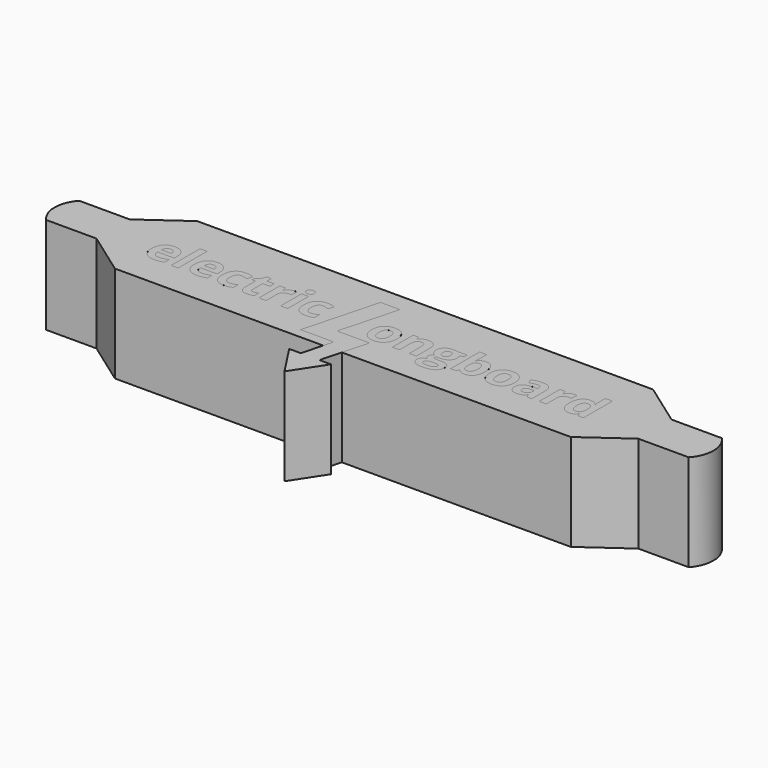
from build123d import *

# Parameters (mm, degrees)
F0_W         = 1.8341714676
F0_H         = 9.3594709833
F0_H_2       = 6.7246538383
F1_DEPTH     = 25
F2_DEPTH     = 25
F3_DEPTH     = 25
F4_DEPTH     = 25
F0_TEXT_SIZE = 12.3176258057
F5_DEPTH     = 25


# Not quite as in the source:
# - Text() gives the source's letters only with a copy of the font that has no kerning and outlines rounded to 1/6400 em; it was checked with that copy


with BuildPart() as f1:
    # F0 (on Top) → F1 (new body)
    with BuildSketch(Plane.XY):
        with BuildLine():
            Line((-5.1384238204, -5.5999981016), (0.0308822297, 13.7858465301))
            Line((0.0308822297, 13.7858465301), (5.042217245, 13.7858465301))
            Line((5.042217245, 13.7858465301), (0.9836744241, -1.434432516))
            Line((0.9836744241, -1.434432516), (9.3703576215, -1.434432516))
            Line((9.3703576215, -1.434432516), (7.5798184046, -8.1492825808))
            Line((7.5798184046, -8.1492825808), (66.7315653023, -8.1492825808))
            Line((66.7315653023, -8.1492825808), (77.8353717101, -0.2207219492))
            Line((77.8353717101, -0.2207219492), (90.8519435273, -0.2207219492))
            ThreePointArc((90.8519435273, -0.2207219492), (92.9463269801, 5.1369656589), (90.8519435273, 10.494653267))
            Line((90.8519435273, 10.494653267), (77.8353717101, 10.494653267))
            Line((77.8353717101, 10.494653267), (66.7315653023, 18.4232138986))
            Line((66.7315653023, 18.4232138986), (-51.0450346977, 18.4232138986))
            Line((-51.0450346977, 18.4232138986), (-62.1488411056, 10.494653267))
            Line((-62.1488411056, 10.494653267), (-75.1654129228, 10.494653267))
            ThreePointArc((-75.1654129228, 10.494653267), (-77.2597963755, 5.1369656589), (-75.1654129228, -0.2207219492))
            Line((-75.1654129228, -0.2207219492), (-62.1488411056, -0.2207219492))
            Line((-62.1488411056, -0.2207219492), (-51.0450346977, -8.1492825808))
            Line((-51.0450346977, -8.1492825808), (2.7661361966, -8.1492825808))
            Line((2.7661361966, -8.1492825808), (3.4459121843, -5.5999981016))
            Line((3.4459121843, -5.5999981016), (-5.1384238204, -5.5999981016))
        make_face()
        with BuildLine():
            add(Edge.make_bspline(
                [(-45.9638463726, -0.0038492581), (-46.5104410177, -0.121251629), (-47.2995389209, -0.121251629)],
                knots=[0, 0, 0, 1, 1, 1], degree=2))
            add(Edge.make_bspline(
                [(-47.2995389209, -0.121251629), (-48.922001195, -0.121251629), (-49.8361999853, 0.7756255)],
                knots=[0, 0, 0, 1, 1, 1], degree=2))
            add(Edge.make_bspline(
                [(-49.8361999853, 0.7756255), (-50.7503987756, 1.6725026289), (-50.7503987756, 3.3142111934)],
                knots=[0, 0, 0, 1, 1, 1], degree=2))
            add(Edge.make_bspline(
                [(-50.7503987756, 3.3142111934), (-50.7503987756, 5.0040354836), (-49.9054866305, 5.9268951045)],
                knots=[0, 0, 0, 1, 1, 1], degree=2))
            add(Edge.make_bspline(
                [(-49.9054866305, 5.9268951045), (-49.0605744853, 6.8497547254), (-47.5689869854, 6.8497547254)],
                knots=[0, 0, 0, 1, 1, 1], degree=2))
            add(Edge.make_bspline(
                [(-47.5689869854, 6.8497547254), (-46.1447615016, 6.8497547254), (-45.3508520259, 6.0385235884)],
                knots=[0, 0, 0, 1, 1, 1], degree=2))
            add(Edge.make_bspline(
                [(-45.3508520259, 6.0385235884), (-44.5569425501, 5.2272924513), (-44.5569425501, 3.7953684514)],
                knots=[0, 0, 0, 1, 1, 1], degree=2))
            Line((-44.5569425501, 3.7953684514), (-44.5569425501, 2.9042652095))
            Line((-44.5569425501, 2.9042652095), (-48.8931317595, 2.9042652095))
            add(Edge.make_bspline(
                [(-48.8931317595, 2.9042652095), (-48.862337695, 2.1228658225), (-48.4292961628, 1.6840504031)],
                knots=[0, 0, 0, 1, 1, 1], degree=2))
            add(Edge.make_bspline(
                [(-48.4292961628, 1.6840504031), (-47.9962546306, 1.2452349838), (-47.2148552435, 1.2452349838)],
                knots=[0, 0, 0, 1, 1, 1], degree=2))
            add(Edge.make_bspline(
                [(-47.2148552435, 1.2452349838), (-46.6066724694, 1.2452349838), (-46.0658517113, 1.3712981854)],
                knots=[0, 0, 0, 1, 1, 1], degree=2))
            add(Edge.make_bspline(
                [(-46.0658517113, 1.3712981854), (-45.5250309533, 1.497361387), (-44.9360944694, 1.7745079676)],
                knots=[0, 0, 0, 1, 1, 1], degree=2))
            Line((-44.9360944694, 1.7745079676), (-44.9360944694, 0.3541317419))
            add(Edge.make_bspline(
                [(-44.9360944694, 0.3541317419), (-45.4172517275, 0.1135531129), (-45.9638463726, -0.0038492581)],
                knots=[0, 0, 0, 1, 1, 1], degree=2))
        make_face(mode=Mode.SUBTRACT)
        with BuildLine():
            add(Edge.make_bspline(
                [(-34.9280235023, -0.0038492581), (-35.4746181474, -0.121251629), (-36.2637160506, -0.121251629)],
                knots=[0, 0, 0, 1, 1, 1], degree=2))
            add(Edge.make_bspline(
                [(-36.2637160506, -0.121251629), (-37.8861783247, -0.121251629), (-38.800377115, 0.7756255)],
                knots=[0, 0, 0, 1, 1, 1], degree=2))
            add(Edge.make_bspline(
                [(-38.800377115, 0.7756255), (-39.7145759052, 1.6725026289), (-39.7145759052, 3.3142111934)],
                knots=[0, 0, 0, 1, 1, 1], degree=2))
            add(Edge.make_bspline(
                [(-39.7145759052, 3.3142111934), (-39.7145759052, 5.0040354836), (-38.8696637601, 5.9268951045)],
                knots=[0, 0, 0, 1, 1, 1], degree=2))
            add(Edge.make_bspline(
                [(-38.8696637601, 5.9268951045), (-38.024751615, 6.8497547254), (-36.5331641151, 6.8497547254)],
                knots=[0, 0, 0, 1, 1, 1], degree=2))
            add(Edge.make_bspline(
                [(-36.5331641151, 6.8497547254), (-35.1089386313, 6.8497547254), (-34.3150291556, 6.0385235884)],
                knots=[0, 0, 0, 1, 1, 1], degree=2))
            add(Edge.make_bspline(
                [(-34.3150291556, 6.0385235884), (-33.5211196798, 5.2272924513), (-33.5211196798, 3.7953684514)],
                knots=[0, 0, 0, 1, 1, 1], degree=2))
            Line((-33.5211196798, 3.7953684514), (-33.5211196798, 2.9042652095))
            Line((-33.5211196798, 2.9042652095), (-37.8573088892, 2.9042652095))
            add(Edge.make_bspline(
                [(-37.8573088892, 2.9042652095), (-37.8265148247, 2.1228658225), (-37.3934732925, 1.6840504031)],
                knots=[0, 0, 0, 1, 1, 1], degree=2))
            add(Edge.make_bspline(
                [(-37.3934732925, 1.6840504031), (-36.9604317602, 1.2452349838), (-36.1790323732, 1.2452349838)],
                knots=[0, 0, 0, 1, 1, 1], degree=2))
            add(Edge.make_bspline(
                [(-36.1790323732, 1.2452349838), (-35.570849599, 1.2452349838), (-35.030028841, 1.3712981854)],
                knots=[0, 0, 0, 1, 1, 1], degree=2))
            add(Edge.make_bspline(
                [(-35.030028841, 1.3712981854), (-34.489208083, 1.497361387), (-33.9002715991, 1.7745079676)],
                knots=[0, 0, 0, 1, 1, 1], degree=2))
            Line((-33.9002715991, 1.7745079676), (-33.9002715991, 0.3541317419))
            add(Edge.make_bspline(
                [(-33.9002715991, 0.3541317419), (-34.3814288572, 0.1135531129), (-34.9280235023, -0.0038492581)],
                knots=[0, 0, 0, 1, 1, 1], degree=2))
        make_face(mode=Mode.SUBTRACT)
        with Locations((-42.1482693164, 4.6797354917)):
            Rectangle(F0_W, F0_H, mode=Mode.SUBTRACT)
        with BuildLine():
            add(Edge.make_bspline(
                [(-28.1533293091, -0.0125100887), (-28.6075417607, -0.121251629), (-29.2984835833, -0.121251629)],
                knots=[0, 0, 0, 1, 1, 1], degree=2))
            add(Edge.make_bspline(
                [(-29.2984835833, -0.121251629), (-32.4375535347, -0.121251629), (-32.4375535347, 3.3257589675)],
                knots=[0, 0, 0, 1, 1, 1], degree=2))
            add(Edge.make_bspline(
                [(-32.4375535347, 3.3257589675), (-32.4375535347, 5.0406034352), (-31.5839805589, 5.9451790803)],
                knots=[0, 0, 0, 1, 1, 1], degree=2))
            add(Edge.make_bspline(
                [(-31.5839805589, 5.9451790803), (-30.7304075832, 6.8497547254), (-29.1368147446, 6.8497547254)],
                knots=[0, 0, 0, 1, 1, 1], degree=2))
            add(Edge.make_bspline(
                [(-29.1368147446, 6.8497547254), (-27.9704895511, 6.8497547254), (-27.0428183576, 6.3936176448)],
                knots=[0, 0, 0, 1, 1, 1], degree=2))
            Line((-27.0428183576, 6.3936176448), (-27.5855637447, 4.9732414191))
            add(Edge.make_bspline(
                [(-27.5855637447, 4.9732414191), (-28.0186052769, 5.148382661), (-28.3910209946, 5.2600111449)],
                knots=[0, 0, 0, 1, 1, 1], degree=2))
            add(Edge.make_bspline(
                [(-28.3910209946, 5.2600111449), (-28.7634367123, 5.3716396287), (-29.1368147446, 5.3716396287)],
                knots=[0, 0, 0, 1, 1, 1], degree=2))
            add(Edge.make_bspline(
                [(-29.1368147446, 5.3716396287), (-30.5687387445, 5.3716396287), (-30.5687387445, 3.3373067417)],
                knots=[0, 0, 0, 1, 1, 1], degree=2))
            add(Edge.make_bspline(
                [(-30.5687387445, 3.3373067417), (-30.5687387445, 1.3645619838), (-29.1368147446, 1.3645619838)],
                knots=[0, 0, 0, 1, 1, 1], degree=2))
            add(Edge.make_bspline(
                [(-29.1368147446, 1.3645619838), (-28.6075417607, 1.3645619838), (-28.1562162527, 1.5060222177)],
                knots=[0, 0, 0, 1, 1, 1], degree=2))
            add(Edge.make_bspline(
                [(-28.1562162527, 1.5060222177), (-27.7048907446, 1.6474824515), (-27.2545275511, 1.9496492096)],
                knots=[0, 0, 0, 1, 1, 1], degree=2))
            Line((-27.2545275511, 1.9496492096), (-27.2545275511, 0.3791519193))
            add(Edge.make_bspline(
                [(-27.2545275511, 0.3791519193), (-27.6991168575, 0.0962314516), (-28.1533293091, -0.0125100887)],
                knots=[0, 0, 0, 1, 1, 1], degree=2))
        make_face(mode=Mode.SUBTRACT)
        with BuildLine():
            add(Edge.make_bspline(
                [(-23.4437620675, 1.5281554515), (-23.2243543578, 1.3414664354), (-22.8625240998, 1.3414664354)],
                knots=[0, 0, 0, 1, 1, 1], degree=2))
            add(Edge.make_bspline(
                [(-22.8625240998, 1.3414664354), (-22.3813668417, 1.3414664354), (-21.7077466805, 1.5512509999)],
                knots=[0, 0, 0, 1, 1, 1], degree=2))
            Line((-21.7077466805, 1.5512509999), (-21.7077466805, 0.1866890161))
            add(Edge.make_bspline(
                [(-21.7077466805, 0.1866890161), (-22.3929146159, -0.121251629), (-23.3917970836, -0.121251629)],
                knots=[0, 0, 0, 1, 1, 1], degree=2))
            add(Edge.make_bspline(
                [(-23.3917970836, -0.121251629), (-24.49268489, -0.121251629), (-24.9950130674, 0.4359284758)],
                knots=[0, 0, 0, 1, 1, 1], degree=2))
            add(Edge.make_bspline(
                [(-24.9950130674, 0.4359284758), (-25.4973412448, 0.9931085806), (-25.4973412448, 2.1055441612)],
                knots=[0, 0, 0, 1, 1, 1], degree=2))
            Line((-25.4973412448, 2.1055441612), (-25.4973412448, 5.3466194513))
            Line((-25.4973412448, 5.3466194513), (-26.3749720834, 5.3466194513))
            Line((-26.3749720834, 5.3466194513), (-26.3749720834, 6.1222449513))
            Line((-26.3749720834, 6.1222449513), (-25.3645418416, 6.7362016125))
            Line((-25.3645418416, 6.7362016125), (-24.8352688577, 8.1565778382))
            Line((-24.8352688577, 8.1565778382), (-23.6631697771, 8.1565778382))
            Line((-23.6631697771, 8.1565778382), (-23.6631697771, 6.7246538383))
            Line((-23.6631697771, 6.7246538383), (-21.7808825837, 6.7246538383))
            Line((-21.7808825837, 6.7246538383), (-21.7808825837, 5.3466194513))
            Line((-21.7808825837, 5.3466194513), (-23.6631697771, 5.3466194513))
            Line((-23.6631697771, 5.3466194513), (-23.6631697771, 2.1055441612))
            add(Edge.make_bspline(
                [(-23.6631697771, 2.1055441612), (-23.6631697771, 1.7148444676), (-23.4437620675, 1.5281554515)],
                knots=[0, 0, 0, 1, 1, 1], degree=2))
        make_face(mode=Mode.SUBTRACT)
        with BuildLine():
            add(Edge.make_bspline(
                [(-17.7535963339, 6.5042838141), (-17.2214364065, 6.8497547254), (-16.5959319711, 6.8497547254)],
                knots=[0, 0, 0, 1, 1, 1], degree=2))
            add(Edge.make_bspline(
                [(-16.5959319711, 6.8497547254), (-16.2225539389, 6.8497547254), (-15.9762014227, 6.7958651125)],
                knots=[0, 0, 0, 1, 1, 1], degree=2))
            Line((-15.9762014227, 6.7958651125), (-16.1147747131, 5.0771713868))
            add(Edge.make_bspline(
                [(-16.1147747131, 5.0771713868), (-16.3380316808, 5.1368348868), (-16.6555954711, 5.1368348868)],
                knots=[0, 0, 0, 1, 1, 1], degree=2))
            add(Edge.make_bspline(
                [(-16.6555954711, 5.1368348868), (-17.5332263098, 5.1368348868), (-18.0240067129, 4.6855093788)],
                knots=[0, 0, 0, 1, 1, 1], degree=2))
            add(Edge.make_bspline(
                [(-18.0240067129, 4.6855093788), (-18.5147871161, 4.2341838707), (-18.5147871161, 3.4219904192)],
                knots=[0, 0, 0, 1, 1, 1], degree=2))
            Line((-18.5147871161, 3.4219904192), (-18.5147871161, 0))
            Line((-18.5147871161, 0), (-20.3489585838, 0))
            Line((-20.3489585838, 0), (-20.3489585838, 6.7246538383))
            Line((-20.3489585838, 6.7246538383), (-18.9593764226, 6.7246538383))
            Line((-18.9593764226, 6.7246538383), (-18.688003729, 5.5929719674))
            Line((-18.688003729, 5.5929719674), (-18.5994707936, 5.5929719674))
            add(Edge.make_bspline(
                [(-18.5994707936, 5.5929719674), (-18.2857562613, 6.1588129029), (-17.7535963339, 6.5042838141)],
                knots=[0, 0, 0, 1, 1, 1], degree=2))
        make_face(mode=Mode.SUBTRACT)
        with Locations((-13.8389008825, 3.3623269192)):
            Rectangle(F0_W, F0_H_2, mode=Mode.SUBTRACT)
        with BuildLine():
            add(Edge.make_bspline(
                [(-7.1209832458, -0.0125100887), (-7.5751956974, -0.121251629), (-8.26613752, -0.121251629)],
                knots=[0, 0, 0, 1, 1, 1], degree=2))
            add(Edge.make_bspline(
                [(-8.26613752, -0.121251629), (-11.4052074714, -0.121251629), (-11.4052074714, 3.3257589675)],
                knots=[0, 0, 0, 1, 1, 1], degree=2))
            add(Edge.make_bspline(
                [(-11.4052074714, 3.3257589675), (-11.4052074714, 5.0406034352), (-10.5516344956, 5.9451790803)],
                knots=[0, 0, 0, 1, 1, 1], degree=2))
            add(Edge.make_bspline(
                [(-10.5516344956, 5.9451790803), (-9.6980615199, 6.8497547254), (-8.1044686813, 6.8497547254)],
                knots=[0, 0, 0, 1, 1, 1], degree=2))
            add(Edge.make_bspline(
                [(-8.1044686813, 6.8497547254), (-6.9381434878, 6.8497547254), (-6.0104722943, 6.3936176448)],
                knots=[0, 0, 0, 1, 1, 1], degree=2))
            Line((-6.0104722943, 6.3936176448), (-6.5532176814, 4.9732414191))
            add(Edge.make_bspline(
                [(-6.5532176814, 4.9732414191), (-6.9862592136, 5.148382661), (-7.3586749313, 5.2600111449)],
                knots=[0, 0, 0, 1, 1, 1], degree=2))
            add(Edge.make_bspline(
                [(-7.3586749313, 5.2600111449), (-7.731090649, 5.3716396287), (-8.1044686813, 5.3716396287)],
                knots=[0, 0, 0, 1, 1, 1], degree=2))
            add(Edge.make_bspline(
                [(-8.1044686813, 5.3716396287), (-9.5363926812, 5.3716396287), (-9.5363926812, 3.3373067417)],
                knots=[0, 0, 0, 1, 1, 1], degree=2))
            add(Edge.make_bspline(
                [(-9.5363926812, 3.3373067417), (-9.5363926812, 1.3645619838), (-8.1044686813, 1.3645619838)],
                knots=[0, 0, 0, 1, 1, 1], degree=2))
            add(Edge.make_bspline(
                [(-8.1044686813, 1.3645619838), (-7.5751956974, 1.3645619838), (-7.1238701894, 1.5060222177)],
                knots=[0, 0, 0, 1, 1, 1], degree=2))
            add(Edge.make_bspline(
                [(-7.1238701894, 1.5060222177), (-6.6725446814, 1.6474824515), (-6.2221814878, 1.9496492096)],
                knots=[0, 0, 0, 1, 1, 1], degree=2))
            Line((-6.2221814878, 1.9496492096), (-6.2221814878, 0.3791519193))
            add(Edge.make_bspline(
                [(-6.2221814878, 0.3791519193), (-6.6667707943, 0.0962314516), (-7.1209832458, -0.0125100887)],
                knots=[0, 0, 0, 1, 1, 1], degree=2))
        make_face(mode=Mode.SUBTRACT)
        with BuildLine():
            add(Edge.make_bspline(
                [(-13.836013939, 7.5599428383), (-14.8348964067, 7.5599428383), (-14.8348964067, 8.4625938543)],
                knots=[0, 0, 0, 1, 1, 1], degree=2))
            add(Edge.make_bspline(
                [(-14.8348964067, 8.4625938543), (-14.8348964067, 9.3594709833), (-13.836013939, 9.3594709833)],
                knots=[0, 0, 0, 1, 1, 1], degree=2))
            add(Edge.make_bspline(
                [(-13.836013939, 9.3594709833), (-12.8371314713, 9.3594709833), (-12.8371314713, 8.4625938543)],
                knots=[0, 0, 0, 1, 1, 1], degree=2))
            add(Edge.make_bspline(
                [(-12.8371314713, 8.4625938543), (-12.8371314713, 8.0353262092), (-13.086370931, 7.7976345237)],
                knots=[0, 0, 0, 1, 1, 1], degree=2))
            add(Edge.make_bspline(
                [(-13.086370931, 7.7976345237), (-13.3356103906, 7.5599428383), (-13.836013939, 7.5599428383)],
                knots=[0, 0, 0, 1, 1, 1], degree=2))
        make_face(mode=Mode.SUBTRACT)
        with BuildLine():
            Line((25.7141219699, 6.7246538383), (28.0602447601, 6.7246538383))
            Line((28.0602447601, 6.7246538383), (28.0602447601, 5.7912087577))
            Line((28.0602447601, 5.7912087577), (27.0074726795, 5.5217606932))
            add(Edge.make_bspline(
                [(27.0074726795, 5.5217606932), (27.2961670344, 5.0694728707), (27.2961670344, 4.5113304514)],
                knots=[0, 0, 0, 1, 1, 1], degree=2))
            add(Edge.make_bspline(
                [(27.2961670344, 4.5113304514), (27.2961670344, 3.4277643063), (26.5407501392, 2.8234307902)],
                knots=[0, 0, 0, 1, 1, 1], degree=2))
            add(Edge.make_bspline(
                [(26.5407501392, 2.8234307902), (25.7853332441, 2.2190972741), (24.4457914378, 2.2190972741)],
                knots=[0, 0, 0, 1, 1, 1], degree=2))
            Line((24.4457914378, 2.2190972741), (24.1147552442, 2.2383435644))
            Line((24.1147552442, 2.2383435644), (23.8433825507, 2.2672129999))
            add(Edge.make_bspline(
                [(23.8433825507, 2.2672129999), (23.560462083, 2.0516545483), (23.560462083, 1.7860557418)],
                knots=[0, 0, 0, 1, 1, 1], degree=2))
            add(Edge.make_bspline(
                [(23.560462083, 1.7860557418), (23.560462083, 1.3895821612), (24.5708923248, 1.3895821612)],
                knots=[0, 0, 0, 1, 1, 1], degree=2))
            Line((24.5708923248, 1.3895821612), (25.7141219699, 1.3895821612))
            add(Edge.make_bspline(
                [(25.7141219699, 1.3895821612), (26.8207836634, 1.3895821612), (27.4010593166, 0.9141987903)],
                knots=[0, 0, 0, 1, 1, 1], degree=2))
            add(Edge.make_bspline(
                [(27.4010593166, 0.9141987903), (27.9813349698, 0.4388154193), (27.9813349698, -0.481157258)],
                knots=[0, 0, 0, 1, 1, 1], degree=2))
            add(Edge.make_bspline(
                [(27.9813349698, -0.481157258), (27.9813349698, -1.6609548547), (26.9978495344, -2.3105171531)],
                knots=[0, 0, 0, 1, 1, 1], degree=2))
            add(Edge.make_bspline(
                [(26.9978495344, -2.3105171531), (26.014364099, -2.9600794514), (24.1744187442, -2.9600794514)],
                knots=[0, 0, 0, 1, 1, 1], degree=2))
            add(Edge.make_bspline(
                [(24.1744187442, -2.9600794514), (22.7675149217, -2.9600794514), (22.0246081153, -2.4692990482)],
                knots=[0, 0, 0, 1, 1, 1], degree=2))
            add(Edge.make_bspline(
                [(22.0246081153, -2.4692990482), (21.2817013089, -1.978518645), (21.2817013089, -1.0951139193)],
                knots=[0, 0, 0, 1, 1, 1], degree=2))
            add(Edge.make_bspline(
                [(21.2817013089, -1.0951139193), (21.2817013089, -0.4869311451), (21.6608532282, -0.0779474758)],
                knots=[0, 0, 0, 1, 1, 1], degree=2))
            add(Edge.make_bspline(
                [(21.6608532282, -0.0779474758), (22.0400051476, 0.3310361935), (22.7732888088, 0.5061774355)],
                knots=[0, 0, 0, 1, 1, 1], degree=2))
            add(Edge.make_bspline(
                [(22.7732888088, 0.5061774355), (22.4903683411, 0.6255044354), (22.2796214621, 0.898801758)],
                knots=[0, 0, 0, 1, 1, 1], degree=2))
            add(Edge.make_bspline(
                [(22.2796214621, 0.898801758), (22.0688745831, 1.1720990806), (22.0688745831, 1.4800397257)],
                knots=[0, 0, 0, 1, 1, 1], degree=2))
            add(Edge.make_bspline(
                [(22.0688745831, 1.4800397257), (22.0688745831, 1.8649655321), (22.2911692363, 2.1199788789)],
                knots=[0, 0, 0, 1, 1, 1], degree=2))
            add(Edge.make_bspline(
                [(22.2911692363, 2.1199788789), (22.5134638895, 2.3749922257), (22.9349576475, 2.6232693708)],
                knots=[0, 0, 0, 1, 1, 1], degree=2))
            add(Edge.make_bspline(
                [(22.9349576475, 2.6232693708), (22.4056846637, 2.8503755966), (22.0958193895, 3.3555907175)],
                knots=[0, 0, 0, 1, 1, 1], degree=2))
            add(Edge.make_bspline(
                [(22.0958193895, 3.3555907175), (21.7859541153, 3.8608058385), (21.7859541153, 4.547898403)],
                knots=[0, 0, 0, 1, 1, 1], degree=2))
            add(Edge.make_bspline(
                [(21.7859541153, 4.547898403), (21.7859541153, 5.6468615803), (22.5019161153, 6.2483081529)],
                knots=[0, 0, 0, 1, 1, 1], degree=2))
            add(Edge.make_bspline(
                [(22.5019161153, 6.2483081529), (23.2178781152, 6.8497547254), (24.5477967765, 6.8497547254)],
                knots=[0, 0, 0, 1, 1, 1], degree=2))
            add(Edge.make_bspline(
                [(24.5477967765, 6.8497547254), (24.8307172442, 6.8497547254), (25.2185299942, 6.7987520561)],
                knots=[0, 0, 0, 1, 1, 1], degree=2))
            add(Edge.make_bspline(
                [(25.2185299942, 6.7987520561), (25.6063427441, 6.7477493867), (25.7141219699, 6.7246538383)],
                knots=[0, 0, 0, 1, 1, 1], degree=2))
        make_face(mode=Mode.SUBTRACT)
        with BuildLine():
            add(Edge.make_bspline(
                [(12.1993769062, 5.2205562497), (12.5958504868, 4.432420661), (12.5958504868, 3.3738746934)],
                knots=[0, 0, 0, 1, 1, 1], degree=2))
            add(Edge.make_bspline(
                [(12.5958504868, 3.3738746934), (12.5958504868, 1.7321661289), (11.7297674224, 0.80545725)],
                knots=[0, 0, 0, 1, 1, 1], degree=2))
            add(Edge.make_bspline(
                [(11.7297674224, 0.80545725), (10.8636843579, -0.121251629), (9.3182072451, -0.121251629)],
                knots=[0, 0, 0, 1, 1, 1], degree=2))
            add(Edge.make_bspline(
                [(9.3182072451, -0.121251629), (8.3501188419, -0.121251629), (7.6100989791, 0.3031290726)],
                knots=[0, 0, 0, 1, 1, 1], degree=2))
            add(Edge.make_bspline(
                [(7.6100989791, 0.3031290726), (6.8700791162, 0.7275097742), (6.4736055356, 1.5214192499)],
                knots=[0, 0, 0, 1, 1, 1], degree=2))
            add(Edge.make_bspline(
                [(6.4736055356, 1.5214192499), (6.077131955, 2.3153287257), (6.077131955, 3.3738746934)],
                knots=[0, 0, 0, 1, 1, 1], degree=2))
            add(Edge.make_bspline(
                [(6.077131955, 3.3738746934), (6.077131955, 5.0213571449), (6.9364788178, 5.9355559351)],
                knots=[0, 0, 0, 1, 1, 1], degree=2))
            add(Edge.make_bspline(
                [(6.9364788178, 5.9355559351), (7.7958256807, 6.8497547254), (9.3547751967, 6.8497547254)],
                knots=[0, 0, 0, 1, 1, 1], degree=2))
            add(Edge.make_bspline(
                [(9.3547751967, 6.8497547254), (10.3228635999, 6.8497547254), (11.0628834627, 6.4292232819)],
                knots=[0, 0, 0, 1, 1, 1], degree=2))
            add(Edge.make_bspline(
                [(11.0628834627, 6.4292232819), (11.8029033256, 6.0086918384), (12.1993769062, 5.2205562497)],
                knots=[0, 0, 0, 1, 1, 1], degree=2))
        make_face(mode=Mode.SUBTRACT)
        with BuildLine():
            Line((20.3193867928, 4.3843049352), (20.3193867928, 0))
            Line((20.3193867928, 0), (18.4852153252, 0))
            Line((18.4852153252, 0), (18.4852153252, 3.9281678546))
            add(Edge.make_bspline(
                [(18.4852153252, 3.9281678546), (18.4852153252, 4.6556776288), (18.2263527204, 5.0194325158)],
                knots=[0, 0, 0, 1, 1, 1], degree=2))
            add(Edge.make_bspline(
                [(18.2263527204, 5.0194325158), (17.9674901156, 5.3831874029), (17.4016491801, 5.3831874029)],
                knots=[0, 0, 0, 1, 1, 1], degree=2))
            add(Edge.make_bspline(
                [(17.4016491801, 5.3831874029), (16.6317975672, 5.3831874029), (16.2892135995, 4.8693114513)],
                knots=[0, 0, 0, 1, 1, 1], degree=2))
            add(Edge.make_bspline(
                [(16.2892135995, 4.8693114513), (15.9466296318, 4.3554354997), (15.9466296318, 3.1640901288)],
                knots=[0, 0, 0, 1, 1, 1], degree=2))
            Line((15.9466296318, 3.1640901288), (15.9466296318, 0))
            Line((15.9466296318, 0), (14.1124581642, 0))
            Line((14.1124581642, 0), (14.1124581642, 6.7246538383))
            Line((14.1124581642, 6.7246538383), (15.5135880996, 6.7246538383))
            Line((15.5135880996, 6.7246538383), (15.7599406157, 5.8643446609))
            Line((15.7599406157, 5.8643446609), (15.8619459544, 5.8643446609))
            add(Edge.make_bspline(
                [(15.8619459544, 5.8643446609), (16.1698865995, 6.3512758061), (16.707820414, 6.6005152657)],
                knots=[0, 0, 0, 1, 1, 1], degree=2))
            add(Edge.make_bspline(
                [(16.707820414, 6.6005152657), (17.2457542285, 6.8497547254), (17.9309221639, 6.8497547254)],
                knots=[0, 0, 0, 1, 1, 1], degree=2))
            add(Edge.make_bspline(
                [(17.9309221639, 6.8497547254), (19.1049458736, 6.8497547254), (19.7121663332, 6.2155894593)],
                knots=[0, 0, 0, 1, 1, 1], degree=2))
            add(Edge.make_bspline(
                [(19.7121663332, 6.2155894593), (20.3193867928, 5.5814241932), (20.3193867928, 4.3843049352)],
                knots=[0, 0, 0, 1, 1, 1], degree=2))
        make_face(mode=Mode.SUBTRACT)
        with BuildLine():
            add(Edge.make_bspline(
                [(31.0010779212, 5.8527968868), (31.645828647, 6.8497547254), (32.9083852921, 6.8497547254)],
                knots=[0, 0, 0, 1, 1, 1], degree=2))
            add(Edge.make_bspline(
                [(32.9083852921, 6.8497547254), (34.099730663, 6.8497547254), (34.7733508243, 5.9211212174)],
                knots=[0, 0, 0, 1, 1, 1], degree=2))
            add(Edge.make_bspline(
                [(34.7733508243, 5.9211212174), (35.4469709855, 4.9924877094), (35.4469709855, 3.3738746934)],
                knots=[0, 0, 0, 1, 1, 1], degree=2))
            add(Edge.make_bspline(
                [(35.4469709855, 3.3738746934), (35.4469709855, 1.7090705805), (34.7521799049, 0.7939094758)],
                knots=[0, 0, 0, 1, 1, 1], degree=2))
            add(Edge.make_bspline(
                [(34.7521799049, 0.7939094758), (34.0573888243, -0.121251629), (32.8602695663, -0.121251629)],
                knots=[0, 0, 0, 1, 1, 1], degree=2))
            add(Edge.make_bspline(
                [(32.8602695663, -0.121251629), (31.6746980825, -0.121251629), (31.0010779212, 0.7390575483)],
                knots=[0, 0, 0, 1, 1, 1], degree=2))
            Line((31.0010779212, 0.7390575483), (30.8759770342, 0.7390575483))
            Line((30.8759770342, 0.7390575483), (30.568036389, 0))
            Line((30.568036389, 0), (29.1669064536, 0))
            Line((29.1669064536, 0), (29.1669064536, 9.3594709833))
            Line((29.1669064536, 9.3594709833), (31.0010779212, 9.3594709833))
            Line((31.0010779212, 9.3594709833), (31.0010779212, 7.1807909189))
            add(Edge.make_bspline(
                [(31.0010779212, 7.1807909189), (31.0010779212, 6.766995677), (30.9298666471, 5.8527968868)],
                knots=[0, 0, 0, 1, 1, 1], degree=2))
            Line((30.9298666471, 5.8527968868), (31.0010779212, 5.8527968868))
        make_face(mode=Mode.SUBTRACT)
        with BuildLine():
            add(Edge.make_bspline(
                [(42.6758776302, 5.2205562497), (43.0723512109, 4.432420661), (43.0723512109, 3.3738746934)],
                knots=[0, 0, 0, 1, 1, 1], degree=2))
            add(Edge.make_bspline(
                [(43.0723512109, 3.3738746934), (43.0723512109, 1.7321661289), (42.2062681464, 0.80545725)],
                knots=[0, 0, 0, 1, 1, 1], degree=2))
            add(Edge.make_bspline(
                [(42.2062681464, 0.80545725), (41.3401850819, -0.121251629), (39.7947079691, -0.121251629)],
                knots=[0, 0, 0, 1, 1, 1], degree=2))
            add(Edge.make_bspline(
                [(39.7947079691, -0.121251629), (38.826619566, -0.121251629), (38.0865997031, 0.3031290726)],
                knots=[0, 0, 0, 1, 1, 1], degree=2))
            add(Edge.make_bspline(
                [(38.0865997031, 0.3031290726), (37.3465798402, 0.7275097742), (36.9501062596, 1.5214192499)],
                knots=[0, 0, 0, 1, 1, 1], degree=2))
            add(Edge.make_bspline(
                [(36.9501062596, 1.5214192499), (36.553632679, 2.3153287257), (36.553632679, 3.3738746934)],
                knots=[0, 0, 0, 1, 1, 1], degree=2))
            add(Edge.make_bspline(
                [(36.553632679, 3.3738746934), (36.553632679, 5.0213571449), (37.4129795418, 5.9355559351)],
                knots=[0, 0, 0, 1, 1, 1], degree=2))
            add(Edge.make_bspline(
                [(37.4129795418, 5.9355559351), (38.2723264047, 6.8497547254), (39.8312759207, 6.8497547254)],
                knots=[0, 0, 0, 1, 1, 1], degree=2))
            add(Edge.make_bspline(
                [(39.8312759207, 6.8497547254), (40.7993643239, 6.8497547254), (41.5393841868, 6.4292232819)],
                knots=[0, 0, 0, 1, 1, 1], degree=2))
            add(Edge.make_bspline(
                [(41.5393841868, 6.4292232819), (42.2794040496, 6.0086918384), (42.6758776302, 5.2205562497)],
                knots=[0, 0, 0, 1, 1, 1], degree=2))
        make_face(mode=Mode.SUBTRACT)
        with BuildLine():
            Line((50.1395890169, 0), (48.8597107105, 0))
            Line((48.8597107105, 0), (48.5036543396, 0.9141987903))
            Line((48.5036543396, 0.9141987903), (48.4555386138, 0.9141987903))
            add(Edge.make_bspline(
                [(48.4555386138, 0.9141987903), (47.9936276461, 0.3310361935), (47.5028472429, 0.1048922823)],
                knots=[0, 0, 0, 1, 1, 1], degree=2))
            add(Edge.make_bspline(
                [(47.5028472429, 0.1048922823), (47.0120668397, -0.121251629), (46.2248935655, -0.121251629)],
                knots=[0, 0, 0, 1, 1, 1], degree=2))
            add(Edge.make_bspline(
                [(46.2248935655, -0.121251629), (45.2568051624, -0.121251629), (44.7005873721, 0.4330415322)],
                knots=[0, 0, 0, 1, 1, 1], degree=2))
            add(Edge.make_bspline(
                [(44.7005873721, 0.4330415322), (44.1443695818, 0.9873346935), (44.1443695818, 2.0093127096)],
                knots=[0, 0, 0, 1, 1, 1], degree=2))
            add(Edge.make_bspline(
                [(44.1443695818, 2.0093127096), (44.1443695818, 3.0794064514), (44.8930502753, 3.5875085159)],
                knots=[0, 0, 0, 1, 1, 1], degree=2))
            add(Edge.make_bspline(
                [(44.8930502753, 3.5875085159), (45.6417309688, 4.0956105804), (47.15064013, 4.1495001933)],
                knots=[0, 0, 0, 1, 1, 1], degree=2))
            Line((47.15064013, 4.1495001933), (48.3188899525, 4.1860681449))
            Line((48.3188899525, 4.1860681449), (48.3188899525, 4.4805363868))
            add(Edge.make_bspline(
                [(48.3188899525, 4.4805363868), (48.3188899525, 5.5025144029), (47.271891759, 5.5025144029)],
                knots=[0, 0, 0, 1, 1, 1], degree=2))
            add(Edge.make_bspline(
                [(47.271891759, 5.5025144029), (46.4654721945, 5.5025144029), (45.3761321623, 5.0155832578)],
                knots=[0, 0, 0, 1, 1, 1], degree=2))
            Line((45.3761321623, 5.0155832578), (44.7698740172, 6.2550443545))
            add(Edge.make_bspline(
                [(44.7698740172, 6.2550443545), (45.9304253236, 6.8632271286), (47.3431030332, 6.8632271286)],
                knots=[0, 0, 0, 1, 1, 1], degree=2))
            add(Edge.make_bspline(
                [(47.3431030332, 6.8632271286), (48.6961172428, 6.8632271286), (49.4178531299, 6.2733283303)],
                knots=[0, 0, 0, 1, 1, 1], degree=2))
            add(Edge.make_bspline(
                [(49.4178531299, 6.2733283303), (50.1395890169, 5.6834295319), (50.1395890169, 4.4805363868)],
                knots=[0, 0, 0, 1, 1, 1], degree=2))
            Line((50.1395890169, 4.4805363868), (50.1395890169, 0))
        make_face(mode=Mode.SUBTRACT)
        with BuildLine():
            add(Edge.make_bspline(
                [(54.6249369763, 6.5042838141), (55.1570969037, 6.8497547254), (55.7826013392, 6.8497547254)],
                knots=[0, 0, 0, 1, 1, 1], degree=2))
            add(Edge.make_bspline(
                [(55.7826013392, 6.8497547254), (56.1559793714, 6.8497547254), (56.4023318875, 6.7958651125)],
                knots=[0, 0, 0, 1, 1, 1], degree=2))
            Line((56.4023318875, 6.7958651125), (56.2637585972, 5.0771713868))
            add(Edge.make_bspline(
                [(56.2637585972, 5.0771713868), (56.0405016295, 5.1368348868), (55.7229378392, 5.1368348868)],
                knots=[0, 0, 0, 1, 1, 1], degree=2))
            add(Edge.make_bspline(
                [(55.7229378392, 5.1368348868), (54.8453070005, 5.1368348868), (54.3545265973, 4.6855093788)],
                knots=[0, 0, 0, 1, 1, 1], degree=2))
            add(Edge.make_bspline(
                [(54.3545265973, 4.6855093788), (53.8637461941, 4.2341838707), (53.8637461941, 3.4219904192)],
                knots=[0, 0, 0, 1, 1, 1], degree=2))
            Line((53.8637461941, 3.4219904192), (53.8637461941, 0))
            Line((53.8637461941, 0), (52.0295747265, 0))
            Line((52.0295747265, 0), (52.0295747265, 6.7246538383))
            Line((52.0295747265, 6.7246538383), (53.4191568877, 6.7246538383))
            Line((53.4191568877, 6.7246538383), (53.6905295812, 5.5929719674))
            Line((53.6905295812, 5.5929719674), (53.7790625167, 5.5929719674))
            add(Edge.make_bspline(
                [(53.7790625167, 5.5929719674), (54.0927770489, 6.1588129029), (54.6249369763, 6.5042838141)],
                knots=[0, 0, 0, 1, 1, 1], degree=2))
        make_face(mode=Mode.SUBTRACT)
        with BuildLine():
            add(Edge.make_bspline(
                [(61.6584937743, 0.8718569516), (61.0329893389, -0.121251629), (59.7511864034, -0.121251629)],
                knots=[0, 0, 0, 1, 1, 1], degree=2))
            add(Edge.make_bspline(
                [(59.7511864034, -0.121251629), (58.5675395487, -0.121251629), (57.8910324439, 0.7996833629)],
                knots=[0, 0, 0, 1, 1, 1], degree=2))
            add(Edge.make_bspline(
                [(57.8910324439, 0.7996833629), (57.2145253391, 1.7206183547), (57.2145253391, 3.350779145)],
                knots=[0, 0, 0, 1, 1, 1], degree=2))
            add(Edge.make_bspline(
                [(57.2145253391, 3.350779145), (57.2145253391, 5.0040354836), (57.9025802181, 5.9268951045)],
                knots=[0, 0, 0, 1, 1, 1], degree=2))
            add(Edge.make_bspline(
                [(57.9025802181, 5.9268951045), (58.5906350971, 6.8497547254), (59.7993021292, 6.8497547254)],
                knots=[0, 0, 0, 1, 1, 1], degree=2))
            add(Edge.make_bspline(
                [(59.7993021292, 6.8497547254), (61.0695572905, 6.8497547254), (61.7374035646, 5.8643446609)],
                knots=[0, 0, 0, 1, 1, 1], degree=2))
            Line((61.7374035646, 5.8643446609), (61.7970670646, 5.8643446609))
            add(Edge.make_bspline(
                [(61.7970670646, 5.8643446609), (61.6584937743, 6.6168746125), (61.6584937743, 7.2058110964)],
                knots=[0, 0, 0, 1, 1, 1], degree=2))
            Line((61.6584937743, 7.2058110964), (61.6584937743, 9.3594709833))
            Line((61.6584937743, 9.3594709833), (63.498439129, 9.3594709833))
            Line((63.498439129, 9.3594709833), (63.498439129, 0))
            Line((63.498439129, 0), (62.0915353065, 0))
            Line((62.0915353065, 0), (61.7374035646, 0.8718569516))
            Line((61.7374035646, 0.8718569516), (61.6584937743, 0.8718569516))
        make_face(mode=Mode.SUBTRACT)
    extrude(amount=F1_DEPTH)


with BuildPart() as f2:
    # F0 (on Top) → F2 (new body)
    with BuildSketch(Plane.XY):
        with BuildLine():
            add(Edge.make_bspline(
                [(8.2712090516, 4.8750853384), (7.9459467452, 4.3785310481), (7.9459467452, 3.3738746934)],
                knots=[0, 0, 0, 1, 1, 1], degree=2))
            add(Edge.make_bspline(
                [(7.9459467452, 3.3738746934), (7.9459467452, 2.3749922257), (8.2740959951, 1.8640032176)],
                knots=[0, 0, 0, 1, 1, 1], degree=2))
            add(Edge.make_bspline(
                [(8.2740959951, 1.8640032176), (8.6022452451, 1.3530142096), (9.3413027935, 1.3530142096)],
                knots=[0, 0, 0, 1, 1, 1], degree=2))
            add(Edge.make_bspline(
                [(9.3413027935, 1.3530142096), (10.0765110838, 1.3530142096), (10.3979241321, 1.8611162741)],
                knots=[0, 0, 0, 1, 1, 1], degree=2))
            add(Edge.make_bspline(
                [(10.3979241321, 1.8611162741), (10.7193371805, 2.3692183386), (10.7193371805, 3.3738746934)],
                knots=[0, 0, 0, 1, 1, 1], degree=2))
            add(Edge.make_bspline(
                [(10.7193371805, 3.3738746934), (10.7193371805, 4.372757161), (10.3950371886, 4.8721983949)],
                knots=[0, 0, 0, 1, 1, 1], degree=2))
            add(Edge.make_bspline(
                [(10.3950371886, 4.8721983949), (10.0707371967, 5.3716396287), (9.3297550193, 5.3716396287)],
                knots=[0, 0, 0, 1, 1, 1], degree=2))
            add(Edge.make_bspline(
                [(9.3297550193, 5.3716396287), (8.596471358, 5.3716396287), (8.2712090516, 4.8750853384)],
                knots=[0, 0, 0, 1, 1, 1], degree=2))
        make_face()
    extrude(amount=F2_DEPTH)


with BuildPart() as f2b:
    # F0 (on Top) → F2, piece 2 (new body)
    with BuildSketch(Plane.XY):
        with BuildLine():
            add(Edge.make_bspline(
                [(33.2394214856, 4.8866331126), (32.902611405, 5.3831874029), (32.3194488083, 5.3831874029)],
                knots=[0, 0, 0, 1, 1, 1], degree=2))
            add(Edge.make_bspline(
                [(32.3194488083, 5.3831874029), (31.6381301309, 5.3831874029), (31.3253779132, 4.9655429029)],
                knots=[0, 0, 0, 1, 1, 1], degree=2))
            add(Edge.make_bspline(
                [(31.3253779132, 4.9655429029), (31.0126256954, 4.547898403), (31.0010779212, 3.5855838869)],
                knots=[0, 0, 0, 1, 1, 1], degree=2))
            Line((31.0010779212, 3.5855838869), (31.0010779212, 3.3854224675))
            add(Edge.make_bspline(
                [(31.0010779212, 3.3854224675), (31.0010779212, 2.3037809515), (31.3234532841, 1.8341714676)],
                knots=[0, 0, 0, 1, 1, 1], degree=2))
            add(Edge.make_bspline(
                [(31.3234532841, 1.8341714676), (31.645828647, 1.3645619838), (32.3425443567, 1.3645619838)],
                knots=[0, 0, 0, 1, 1, 1], degree=2))
            add(Edge.make_bspline(
                [(32.3425443567, 1.3645619838), (32.9083852921, 1.3645619838), (33.2423084292, 1.885174137)],
                knots=[0, 0, 0, 1, 1, 1], degree=2))
            add(Edge.make_bspline(
                [(33.2423084292, 1.885174137), (33.5762315663, 2.4057862902), (33.5762315663, 3.3988948708)],
                knots=[0, 0, 0, 1, 1, 1], degree=2))
            add(Edge.make_bspline(
                [(33.5762315663, 3.3988948708), (33.5762315663, 4.3900788223), (33.2394214856, 4.8866331126)],
                knots=[0, 0, 0, 1, 1, 1], degree=2))
        make_face()
    extrude(amount=F2_DEPTH)


with BuildPart() as f3:
    # F0 (on Top) → F3 (new body)
    with BuildSketch(Plane.XY):
        Polygon((5.042217245, 13.7858465301), (0.0308822297, 13.7858465301), (-5.1384238204, -5.5999981016), (3.4459121843, -5.5999981016), (2.7661361966, -8.1492825808), (1.3179426054, -13.5802738369), (-1.6820573946, -13.5802738369), (3.7188784392, -21.8480560623), (9.1189136017, -13.5816525894), (6.1325254744, -13.5768961927), (7.5798184046, -8.1492825808), (9.3703576215, -1.434432516), (0.9836744241, -1.434432516), align=None)
    extrude(amount=F3_DEPTH)


with BuildPart() as f4:
    # F0 (on Top) → F4 (new body)
    with BuildSketch(Plane.XY):
        with BuildLine():
            add(Edge.make_bspline(
                [(24.5477967765, 5.7373191448), (23.5373665346, 5.7373191448), (23.5373665346, 4.5228782255)],
                knots=[0, 0, 0, 1, 1, 1], degree=2))
            add(Edge.make_bspline(
                [(23.5373665346, 4.5228782255), (23.5373665346, 3.9762835804), (23.7866059942, 3.6567951611)],
                knots=[0, 0, 0, 1, 1, 1], degree=2))
            add(Edge.make_bspline(
                [(23.7866059942, 3.6567951611), (24.0358454539, 3.3373067417), (24.5477967765, 3.3373067417)],
                knots=[0, 0, 0, 1, 1, 1], degree=2))
            add(Edge.make_bspline(
                [(24.5477967765, 3.3373067417), (25.0635973571, 3.3373067417), (25.3041759861, 3.6567951611)],
                knots=[0, 0, 0, 1, 1, 1], degree=2))
            add(Edge.make_bspline(
                [(25.3041759861, 3.6567951611), (25.5447546151, 3.9762835804), (25.5447546151, 4.5228782255)],
                knots=[0, 0, 0, 1, 1, 1], degree=2))
            add(Edge.make_bspline(
                [(25.5447546151, 4.5228782255), (25.5447546151, 5.7373191448), (24.5477967765, 5.7373191448)],
                knots=[0, 0, 0, 1, 1, 1], degree=2))
        make_face()
    extrude(amount=F4_DEPTH)


with BuildPart() as f4b:
    # F0 (on Top) → F4, piece 2 (new body)
    with BuildSketch(Plane.XY):
        with BuildLine():
            add(Edge.make_bspline(
                [(23.2092172846, -0.3223753629), (22.8695202604, -0.5600670484), (22.8695202604, -0.9507667419)],
                knots=[0, 0, 0, 1, 1, 1], degree=2))
            add(Edge.make_bspline(
                [(22.8695202604, -0.9507667419), (22.8695202604, -1.3299186612), (23.2332751475, -1.5464394273)],
                knots=[0, 0, 0, 1, 1, 1], degree=2))
            add(Edge.make_bspline(
                [(23.2332751475, -1.5464394273), (23.5970300346, -1.7629601934), (24.2533285345, -1.7629601934)],
                knots=[0, 0, 0, 1, 1, 1], degree=2))
            add(Edge.make_bspline(
                [(24.2533285345, -1.7629601934), (25.238738599, -1.7629601934), (25.7978433328, -1.4915874999)],
                knots=[0, 0, 0, 1, 1, 1], degree=2))
            add(Edge.make_bspline(
                [(25.7978433328, -1.4915874999), (26.3569480667, -1.2202148064), (26.3569480667, -0.7525299516)],
                knots=[0, 0, 0, 1, 1, 1], degree=2))
            add(Edge.make_bspline(
                [(26.3569480667, -0.7525299516), (26.3569480667, -0.3733780322), (26.0268741877, -0.2290308548)],
                knots=[0, 0, 0, 1, 1, 1], degree=2))
            add(Edge.make_bspline(
                [(26.0268741877, -0.2290308548), (25.6968003087, -0.0846836774), (25.0039338571, -0.0846836774)],
                knots=[0, 0, 0, 1, 1, 1], degree=2))
            Line((25.0039338571, -0.0846836774), (24.0531671152, -0.0846836774))
            add(Edge.make_bspline(
                [(24.0531671152, -0.0846836774), (23.5489143088, -0.0846836774), (23.2092172846, -0.3223753629)],
                knots=[0, 0, 0, 1, 1, 1], degree=2))
        make_face()
    extrude(amount=F4_DEPTH)


with BuildPart() as f4c:
    # F0 (on Top) → F4, piece 3 (new body)
    with BuildSketch(Plane.XY):
        with BuildLine():
            add(Edge.make_bspline(
                [(38.7477097756, 4.8750853384), (38.4224474692, 4.3785310481), (38.4224474692, 3.3738746934)],
                knots=[0, 0, 0, 1, 1, 1], degree=2))
            add(Edge.make_bspline(
                [(38.4224474692, 3.3738746934), (38.4224474692, 2.3749922257), (38.7505967192, 1.8640032176)],
                knots=[0, 0, 0, 1, 1, 1], degree=2))
            add(Edge.make_bspline(
                [(38.7505967192, 1.8640032176), (39.0787459692, 1.3530142096), (39.8178035175, 1.3530142096)],
                knots=[0, 0, 0, 1, 1, 1], degree=2))
            add(Edge.make_bspline(
                [(39.8178035175, 1.3530142096), (40.5530118078, 1.3530142096), (40.8744248562, 1.8611162741)],
                knots=[0, 0, 0, 1, 1, 1], degree=2))
            add(Edge.make_bspline(
                [(40.8744248562, 1.8611162741), (41.1958379045, 2.3692183386), (41.1958379045, 3.3738746934)],
                knots=[0, 0, 0, 1, 1, 1], degree=2))
            add(Edge.make_bspline(
                [(41.1958379045, 3.3738746934), (41.1958379045, 4.372757161), (40.8715379126, 4.8721983949)],
                knots=[0, 0, 0, 1, 1, 1], degree=2))
            add(Edge.make_bspline(
                [(40.8715379126, 4.8721983949), (40.5472379207, 5.3716396287), (39.8062557433, 5.3716396287)],
                knots=[0, 0, 0, 1, 1, 1], degree=2))
            add(Edge.make_bspline(
                [(39.8062557433, 5.3716396287), (39.0729720821, 5.3716396287), (38.7477097756, 4.8750853384)],
                knots=[0, 0, 0, 1, 1, 1], degree=2))
        make_face()
    extrude(amount=F4_DEPTH)


with BuildPart() as f4d:
    # F0 (on Top) → F4, piece 4 (new body)
    with BuildSketch(Plane.XY):
        with BuildLine():
            Line((48.3188899525, 2.5616812418), (48.3188899525, 3.115974403))
            Line((48.3188899525, 3.115974403), (47.6087018396, 3.0909542256))
            add(Edge.make_bspline(
                [(47.6087018396, 3.0909542256), (46.8080561623, 3.0678586772), (46.4173564687, 2.8032221853)],
                knots=[0, 0, 0, 1, 1, 1], degree=2))
            add(Edge.make_bspline(
                [(46.4173564687, 2.8032221853), (46.0266567752, 2.5385856934), (46.0266567752, 1.9977649354)],
                knots=[0, 0, 0, 1, 1, 1], degree=2))
            add(Edge.make_bspline(
                [(46.0266567752, 1.9977649354), (46.0266567752, 1.2202148064), (46.9158353881, 1.2202148064)],
                knots=[0, 0, 0, 1, 1, 1], degree=2))
            add(Edge.make_bspline(
                [(46.9158353881, 1.2202148064), (47.5548122267, 1.2202148064), (47.9368510896, 1.5878189515)],
                knots=[0, 0, 0, 1, 1, 1], degree=2))
            add(Edge.make_bspline(
                [(47.9368510896, 1.5878189515), (48.3188899525, 1.9554230967), (48.3188899525, 2.5616812418)],
                knots=[0, 0, 0, 1, 1, 1], degree=2))
        make_face()
    extrude(amount=F4_DEPTH)


with BuildPart() as f4e:
    # F0 (on Top) → F4, piece 5 (new body)
    with BuildSketch(Plane.XY):
        with BuildLine():
            add(Edge.make_bspline(
                [(59.4143763228, 1.8380207257), (59.7569602905, 1.3414664354), (60.3959371292, 1.3414664354)],
                knots=[0, 0, 0, 1, 1, 1], degree=2))
            add(Edge.make_bspline(
                [(60.3959371292, 1.3414664354), (61.0984267259, 1.3414664354), (61.4265759759, 1.7504501047)],
                knots=[0, 0, 0, 1, 1, 1], degree=2))
            add(Edge.make_bspline(
                [(61.4265759759, 1.7504501047), (61.7547252259, 2.1594337741), (61.7855192904, 3.1390699514)],
                knots=[0, 0, 0, 1, 1, 1], degree=2))
            Line((61.7855192904, 3.1390699514), (61.7855192904, 3.3373067417))
            add(Edge.make_bspline(
                [(61.7855192904, 3.3373067417), (61.7855192904, 4.4208728868), (61.4515961533, 4.8895200562)],
                knots=[0, 0, 0, 1, 1, 1], degree=2))
            add(Edge.make_bspline(
                [(61.4515961533, 4.8895200562), (61.1176730163, 5.3581672255), (60.3651430647, 5.3581672255)],
                knots=[0, 0, 0, 1, 1, 1], degree=2))
            add(Edge.make_bspline(
                [(60.3651430647, 5.3581672255), (59.7511864034, 5.3581672255), (59.4114893793, 4.8385173868)],
                knots=[0, 0, 0, 1, 1, 1], degree=2))
            add(Edge.make_bspline(
                [(59.4114893793, 4.8385173868), (59.0717923551, 4.3188675481), (59.0717923551, 3.3257589675)],
                knots=[0, 0, 0, 1, 1, 1], degree=2))
            add(Edge.make_bspline(
                [(59.0717923551, 3.3257589675), (59.0717923551, 2.334575016), (59.4143763228, 1.8380207257)],
                knots=[0, 0, 0, 1, 1, 1], degree=2))
        make_face()
    extrude(amount=F4_DEPTH)


with BuildPart() as f4f:
    # F0 (on Top) → F4, piece 6 (new body)
    with BuildSketch(Plane.XY):
        with BuildLine():
            add(Edge.make_bspline(
                [(-46.6316926468, 5.1753274674), (-46.9742766145, 5.5448562416), (-47.5574392112, 5.5448562416)],
                knots=[0, 0, 0, 1, 1, 1], degree=2))
            add(Edge.make_bspline(
                [(-47.5574392112, 5.5448562416), (-48.140601808, 5.5448562416), (-48.4716380015, 5.1753274674)],
                knots=[0, 0, 0, 1, 1, 1], degree=2))
            add(Edge.make_bspline(
                [(-48.4716380015, 5.1753274674), (-48.802674195, 4.8057986933), (-48.8507899208, 4.1264046449)],
                knots=[0, 0, 0, 1, 1, 1], degree=2))
            Line((-48.8507899208, 4.1264046449), (-46.2756362758, 4.1264046449))
            add(Edge.make_bspline(
                [(-46.2756362758, 4.1264046449), (-46.289108679, 4.8057986933), (-46.6316926468, 5.1753274674)],
                knots=[0, 0, 0, 1, 1, 1], degree=2))
        make_face()
    extrude(amount=F4_DEPTH)


with BuildPart() as f4g:
    # F0 (on Top) → F4, piece 7 (new body)
    with BuildSketch(Plane.XY):
        with BuildLine():
            add(Edge.make_bspline(
                [(-35.5958697764, 5.1753274674), (-35.9384537442, 5.5448562416), (-36.5216163409, 5.5448562416)],
                knots=[0, 0, 0, 1, 1, 1], degree=2))
            add(Edge.make_bspline(
                [(-36.5216163409, 5.5448562416), (-37.1047789376, 5.5448562416), (-37.4358151312, 5.1753274674)],
                knots=[0, 0, 0, 1, 1, 1], degree=2))
            add(Edge.make_bspline(
                [(-37.4358151312, 5.1753274674), (-37.7668513247, 4.8057986933), (-37.8149670505, 4.1264046449)],
                knots=[0, 0, 0, 1, 1, 1], degree=2))
            Line((-37.8149670505, 4.1264046449), (-35.2398134055, 4.1264046449))
            add(Edge.make_bspline(
                [(-35.2398134055, 4.1264046449), (-35.2532858087, 4.8057986933), (-35.5958697764, 5.1753274674)],
                knots=[0, 0, 0, 1, 1, 1], degree=2))
        make_face()
    extrude(amount=F4_DEPTH)


with BuildPart() as f5:
    # F0 (on Top) → F5 (new body)
    with BuildSketch(Plane.XY):
        with Locations((-51.3046919368, 0)):
            Text('electric', F0_TEXT_SIZE, font='Open Sans', font_style=FontStyle.BOLD, text_align=(TextAlign.LEFT, TextAlign.BOTTOM))
        with Locations((5.5228387937, 0)):
            Text('ongboard', F0_TEXT_SIZE, font='Open Sans', font_style=FontStyle.BOLD, text_align=(TextAlign.LEFT, TextAlign.BOTTOM))
    extrude(amount=F5_DEPTH)


solid = Compound([f1.part, f2.part, f2b.part, f3.part, f4.part, f4b.part, f4c.part, f4d.part, f4e.part, f4f.part, f4g.part, f5.part])
